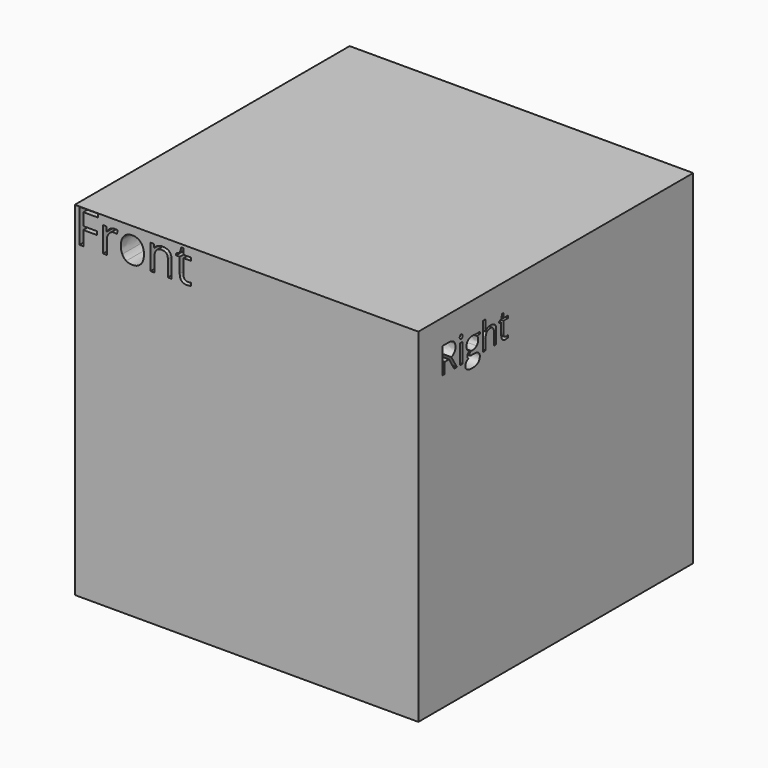
from build123d import *

# Parameters (mm, degrees)
F0_W     = 150
F0_H     = 150
F2_DEPTH = 75
F1_W     = 150
F1_H     = 150
F1_W_2   = 1.2864061088
F1_H_2   = 8.4892888683
F3_DEPTH = 75


with BuildPart() as f2:
    # F0 (on Front) → F2 (new body, symmetric)
    with BuildSketch(Plane.XZ):
        Rectangle(F0_W, F0_H)
        Polygon((-71.2858654449, 66.4917797723), (-71.2858654449, 60.2331906557), (-72.9875094904, 60.2331906557), (-72.9875094904, 74.8750204938), (-64.8253863567, 74.8750204938), (-64.8253863567, 73.3624480089), (-71.2858654449, 73.3624480089), (-71.2858654449, 68.0043522573), (-65.2163478889, 68.0043522573), (-65.2163478889, 66.4917797723), align=None, mode=Mode.SUBTRACT)
        with BuildLine():
            add(Edge.make_bspline(
                [(-59.537791865, 70.8292095569), (-58.6757537327, 71.410844951), (-57.6438716561, 71.410844951)],
                knots=[0, 0, 0, 1, 1, 1], degree=2))
            add(Edge.make_bspline(
                [(-57.6438716561, 71.410844951), (-56.9132222354, 71.410844951), (-56.3331891427, 71.2890700476)],
                knots=[0, 0, 0, 1, 1, 1], degree=2))
            Line((-56.3331891427, 71.2890700476), (-56.5639205387, 69.7476561382))
            add(Edge.make_bspline(
                [(-56.5639205387, 69.7476561382), (-57.2432963158, 69.8982724661), (-57.7656465595, 69.8982724661)],
                knots=[0, 0, 0, 1, 1, 1], degree=2))
            add(Edge.make_bspline(
                [(-57.7656465595, 69.8982724661), (-59.098761292, 69.8982724661), (-60.0441190951, 68.8167190474)],
                knots=[0, 0, 0, 1, 1, 1], degree=2))
            add(Edge.make_bspline(
                [(-60.0441190951, 68.8167190474), (-60.9894768982, 67.7351656286), (-60.9894768982, 66.1232504593)],
                knots=[0, 0, 0, 1, 1, 1], degree=2))
            Line((-60.9894768982, 66.1232504593), (-60.9894768982, 60.2331906557))
            Line((-60.9894768982, 60.2331906557), (-62.652665711, 60.2331906557))
            Line((-62.652665711, 60.2331906557), (-62.652665711, 71.2089549795))
            Line((-62.652665711, 71.2089549795), (-61.2810957459, 71.2089549795))
            Line((-61.2810957459, 71.2089549795), (-61.0888195826, 69.1772368536))
            Line((-61.0888195826, 69.1772368536), (-61.0087045145, 69.1772368536))
            add(Edge.make_bspline(
                [(-61.0087045145, 69.1772368536), (-60.3998299973, 70.2475741629), (-59.537791865, 70.8292095569)],
                knots=[0, 0, 0, 1, 1, 1], degree=2))
        make_face(mode=Mode.SUBTRACT)
        with BuildLine():
            add(Edge.make_bspline(
                [(-46.1633824035, 69.8774425484), (-44.8062331506, 68.3440401458), (-44.8062331506, 65.7322889272)],
                knots=[0, 0, 0, 1, 1, 1], degree=2))
            add(Edge.make_bspline(
                [(-44.8062331506, 65.7322889272), (-44.8062331506, 63.0468318459), (-46.1569731981, 61.539066265)],
                knots=[0, 0, 0, 1, 1, 1], degree=2))
            add(Edge.make_bspline(
                [(-46.1569731981, 61.539066265), (-47.5077132455, 60.0313006842), (-49.8919376709, 60.0313006842)],
                knots=[0, 0, 0, 1, 1, 1], degree=2))
            add(Edge.make_bspline(
                [(-49.8919376709, 60.0313006842), (-51.3660549231, 60.0313006842), (-52.5068934923, 60.7234948722)],
                knots=[0, 0, 0, 1, 1, 1], degree=2))
            add(Edge.make_bspline(
                [(-52.5068934923, 60.7234948722), (-53.6477320614, 61.4156890602), (-54.2694249895, 62.7071439573)],
                knots=[0, 0, 0, 1, 1, 1], degree=2))
            add(Edge.make_bspline(
                [(-54.2694249895, 62.7071439573), (-54.8911179177, 63.9985988544), (-54.8911179177, 65.7322889272)],
                knots=[0, 0, 0, 1, 1, 1], degree=2))
            add(Edge.make_bspline(
                [(-54.8911179177, 65.7322889272), (-54.8911179177, 68.4145414057), (-53.548389377, 69.9126931784)],
                knots=[0, 0, 0, 1, 1, 1], degree=2))
            add(Edge.make_bspline(
                [(-53.548389377, 69.9126931784), (-52.2056608364, 71.410844951), (-49.821436411, 71.410844951)],
                knots=[0, 0, 0, 1, 1, 1], degree=2))
            add(Edge.make_bspline(
                [(-49.821436411, 71.410844951), (-47.5205316564, 71.410844951), (-46.1633824035, 69.8774425484)],
                knots=[0, 0, 0, 1, 1, 1], degree=2))
        make_face(mode=Mode.SUBTRACT)
        with BuildLine():
            Line((-32.7152670794, 60.2331906557), (-34.3784558923, 60.2331906557))
            Line((-34.3784558923, 60.2331906557), (-34.3784558923, 67.3345902883))
            add(Edge.make_bspline(
                [(-34.3784558923, 67.3345902883), (-34.3784558923, 68.6741142262), (-34.9889327109, 69.3358646884)],
                knots=[0, 0, 0, 1, 1, 1], degree=2))
            add(Edge.make_bspline(
                [(-34.9889327109, 69.3358646884), (-35.5994095295, 69.9976151505), (-36.9036828375, 69.9976151505)],
                knots=[0, 0, 0, 1, 1, 1], degree=2))
            add(Edge.make_bspline(
                [(-36.9036828375, 69.9976151505), (-38.6245544993, 69.9976151505), (-39.4257051799, 69.0666780597)],
                knots=[0, 0, 0, 1, 1, 1], degree=2))
            add(Edge.make_bspline(
                [(-39.4257051799, 69.0666780597), (-40.2268558605, 68.1357409689), (-40.2268558605, 65.9918617477)],
                knots=[0, 0, 0, 1, 1, 1], degree=2))
            Line((-40.2268558605, 65.9918617477), (-40.2268558605, 60.2331906557))
            Line((-40.2268558605, 60.2331906557), (-41.8900446733, 60.2331906557))
            Line((-41.8900446733, 60.2331906557), (-41.8900446733, 71.2089549795))
            Line((-41.8900446733, 71.2089549795), (-40.5377023245, 71.2089549795))
            Line((-40.5377023245, 71.2089549795), (-40.2685156959, 69.7059963028))
            Line((-40.2685156959, 69.7059963028), (-40.1884006278, 69.7059963028))
            add(Edge.make_bspline(
                [(-40.1884006278, 69.7059963028), (-39.6756641922, 70.5167607915), (-38.7543409096, 70.9638028713)],
                knots=[0, 0, 0, 1, 1, 1], degree=2))
            add(Edge.make_bspline(
                [(-38.7543409096, 70.9638028713), (-37.8330176269, 71.410844951), (-36.701792866, 71.410844951)],
                knots=[0, 0, 0, 1, 1, 1], degree=2))
            add(Edge.make_bspline(
                [(-36.701792866, 71.410844951), (-34.7181437809, 71.410844951), (-33.7167054302, 70.4542710384)],
                knots=[0, 0, 0, 1, 1, 1], degree=2))
            add(Edge.make_bspline(
                [(-33.7167054302, 70.4542710384), (-32.7152670794, 69.4976971258), (-32.7152670794, 67.3922731373)],
                knots=[0, 0, 0, 1, 1, 1], degree=2))
            Line((-32.7152670794, 67.3922731373), (-32.7152670794, 60.2331906557))
        make_face(mode=Mode.SUBTRACT)
        with BuildLine():
            add(Edge.make_bspline(
                [(-27.0495294664, 61.9364370026), (-26.5784528663, 61.4060752521), (-25.7580745694, 61.4060752521)],
                knots=[0, 0, 0, 1, 1, 1], degree=2))
            add(Edge.make_bspline(
                [(-25.7580745694, 61.4060752521), (-25.3158393937, 61.4060752521), (-24.9056502452, 61.4701673065)],
                knots=[0, 0, 0, 1, 1, 1], degree=2))
            add(Edge.make_bspline(
                [(-24.9056502452, 61.4701673065), (-24.4954610968, 61.534259361), (-24.2551158926, 61.6047606208)],
                knots=[0, 0, 0, 1, 1, 1], degree=2))
            Line((-24.2551158926, 61.6047606208), (-24.2551158926, 60.3325333401))
            add(Edge.make_bspline(
                [(-24.2551158926, 60.3325333401), (-24.5243025213, 60.2043492312), (-25.0498573677, 60.1178249577)],
                knots=[0, 0, 0, 1, 1, 1], degree=2))
            add(Edge.make_bspline(
                [(-25.0498573677, 60.1178249577), (-25.5754122142, 60.0313006842), (-25.9984197735, 60.0313006842)],
                knots=[0, 0, 0, 1, 1, 1], degree=2))
            add(Edge.make_bspline(
                [(-25.9984197735, 60.0313006842), (-29.1805902768, 60.0313006842), (-29.1805902768, 63.3865197344)],
                knots=[0, 0, 0, 1, 1, 1], degree=2))
            Line((-29.1805902768, 63.3865197344), (-29.1805902768, 69.9175000825))
            Line((-29.1805902768, 69.9175000825), (-30.7540502134, 69.9175000825))
            Line((-30.7540502134, 69.9175000825), (-30.7540502134, 70.718650763))
            Line((-30.7540502134, 70.718650763), (-29.1805902768, 71.410844951))
            Line((-29.1805902768, 71.410844951), (-28.4819868833, 73.753409541))
            Line((-28.4819868833, 73.753409541), (-27.5206060666, 73.753409541))
            Line((-27.5206060666, 73.753409541), (-27.5206060666, 71.2089549795))
            Line((-27.5206060666, 71.2089549795), (-24.3352309607, 71.2089549795))
            Line((-24.3352309607, 71.2089549795), (-24.3352309607, 69.9175000825))
            Line((-24.3352309607, 69.9175000825), (-27.5206060666, 69.9175000825))
            Line((-27.5206060666, 69.9175000825), (-27.5206060666, 63.4570209943))
            add(Edge.make_bspline(
                [(-27.5206060666, 63.4570209943), (-27.5206060666, 62.4667987531), (-27.0495294664, 61.9364370026)],
                knots=[0, 0, 0, 1, 1, 1], degree=2))
        make_face(mode=Mode.SUBTRACT)
    extrude(amount=F2_DEPTH, both=True)

    # F1 (on Right) → F3 (intersect, symmetric)
    with BuildSketch(Plane.YZ):
        Rectangle(F1_W, F1_H)
        with BuildLine():
            Line((-44.2826830679, 61.3081981557), (-41.3479916751, 61.3081981557))
            Line((-41.3479916751, 61.3081981557), (-41.3479916751, 60.495209324))
            Line((-41.3479916751, 60.495209324), (-42.9194396, 60.3093124874))
            add(Edge.make_bspline(
                [(-42.9194396, 60.3093124874), (-42.7037992696, 60.0391424183), (-42.53277418, 59.6004258841)],
                knots=[0, 0, 0, 1, 1, 1], degree=2))
            add(Edge.make_bspline(
                [(-42.53277418, 59.6004258841), (-42.3617490904, 59.1617093499), (-42.3617490904, 58.6139333383)],
                knots=[0, 0, 0, 1, 1, 1], degree=2))
            add(Edge.make_bspline(
                [(-42.3617490904, 58.6139333383), (-42.3617490904, 57.3647065968), (-43.2143959139, 56.6211192506)],
                knots=[0, 0, 0, 1, 1, 1], degree=2))
            add(Edge.make_bspline(
                [(-43.2143959139, 56.6211192506), (-44.0670427375, 55.8775319045), (-45.5542174297, 55.8775319045)],
                knots=[0, 0, 0, 1, 1, 1], degree=2))
            add(Edge.make_bspline(
                [(-45.5542174297, 55.8775319045), (-45.9334469763, 55.8775319045), (-46.2655826575, 55.9394975167)],
                knots=[0, 0, 0, 1, 1, 1], degree=2))
            add(Edge.make_bspline(
                [(-46.2655826575, 55.9394975167), (-47.0860073627, 55.5057382315), (-47.0860073627, 54.8489027424)],
                knots=[0, 0, 0, 1, 1, 1], degree=2))
            add(Edge.make_bspline(
                [(-47.0860073627, 54.8489027424), (-47.0860073627, 54.4994166897), (-46.7997262345, 54.3333488491)],
                knots=[0, 0, 0, 1, 1, 1], degree=2))
            add(Edge.make_bspline(
                [(-46.7997262345, 54.3333488491), (-46.5134451062, 54.1672810084), (-45.8169516254, 54.1672810084)],
                knots=[0, 0, 0, 1, 1, 1], degree=2))
            Line((-45.8169516254, 54.1672810084), (-44.3149051862, 54.1672810084))
            add(Edge.make_bspline(
                [(-44.3149051862, 54.1672810084), (-42.9343113469, 54.1672810084), (-42.1956812497, 53.5860435662)],
                knots=[0, 0, 0, 1, 1, 1], degree=2))
            add(Edge.make_bspline(
                [(-42.1956812497, 53.5860435662), (-41.4570511526, 53.004806124), (-41.4570511526, 51.8968609783)],
                knots=[0, 0, 0, 1, 1, 1], degree=2))
            add(Edge.make_bspline(
                [(-41.4570511526, 51.8968609783), (-41.4570511526, 50.4865236451), (-42.5873039187, 49.7466542357)],
                knots=[0, 0, 0, 1, 1, 1], degree=2))
            add(Edge.make_bspline(
                [(-42.5873039187, 49.7466542357), (-43.7175566848, 49.0067848263), (-45.886353111, 49.0067848263)],
                knots=[0, 0, 0, 1, 1, 1], degree=2))
            add(Edge.make_bspline(
                [(-45.886353111, 49.0067848263), (-47.5519887663, 49.0067848263), (-48.4542080796, 49.6264409481)],
                knots=[0, 0, 0, 1, 1, 1], degree=2))
            add(Edge.make_bspline(
                [(-48.4542080796, 49.6264409481), (-49.3564273929, 50.2460970699), (-49.3564273929, 51.3788284605)],
                knots=[0, 0, 0, 1, 1, 1], degree=2))
            add(Edge.make_bspline(
                [(-49.3564273929, 51.3788284605), (-49.3564273929, 52.1521593004), (-48.8607024955, 52.7185249957)],
                knots=[0, 0, 0, 1, 1, 1], degree=2))
            add(Edge.make_bspline(
                [(-48.8607024955, 52.7185249957), (-48.3649775981, 53.284890691), (-47.4677155338, 53.4856592745)],
                knots=[0, 0, 0, 1, 1, 1], degree=2))
            add(Edge.make_bspline(
                [(-47.4677155338, 53.4856592745), (-47.7924153416, 53.6318981192), (-48.0130129209, 53.9417261801)],
                knots=[0, 0, 0, 1, 1, 1], degree=2))
            add(Edge.make_bspline(
                [(-48.0130129209, 53.9417261801), (-48.2336105003, 54.251554241), (-48.2336105003, 54.6630059058)],
                knots=[0, 0, 0, 1, 1, 1], degree=2))
            add(Edge.make_bspline(
                [(-48.2336105003, 54.6630059058), (-48.2336105003, 55.1265086849), (-47.9857480516, 55.4759947376)],
                knots=[0, 0, 0, 1, 1, 1], degree=2))
            add(Edge.make_bspline(
                [(-47.9857480516, 55.4759947376), (-47.7378856029, 55.8254807903), (-47.2025027136, 56.1501805981)],
                knots=[0, 0, 0, 1, 1, 1], degree=2))
            add(Edge.make_bspline(
                [(-47.2025027136, 56.1501805981), (-47.8618168272, 56.4203506672), (-48.2757471166, 57.0709895951)],
                knots=[0, 0, 0, 1, 1, 1], degree=2))
            add(Edge.make_bspline(
                [(-48.2757471166, 57.0709895951), (-48.6896774059, 57.7216285229), (-48.6896774059, 58.5594035996)],
                knots=[0, 0, 0, 1, 1, 1], degree=2))
            add(Edge.make_bspline(
                [(-48.6896774059, 58.5594035996), (-48.6896774059, 59.9523905613), (-47.8531416415, 60.7083710299)],
                knots=[0, 0, 0, 1, 1, 1], degree=2))
            add(Edge.make_bspline(
                [(-47.8531416415, 60.7083710299), (-47.0166058771, 61.4643514984), (-45.4848159441, 61.4643514984)],
                knots=[0, 0, 0, 1, 1, 1], degree=2))
            add(Edge.make_bspline(
                [(-45.4848159441, 61.4643514984), (-44.8180659571, 61.4643514984), (-44.2826830679, 61.3081981557)],
                knots=[0, 0, 0, 1, 1, 1], degree=2))
        make_face(mode=Mode.SUBTRACT)
        with BuildLine():
            Line((-58.2398175546, 57.5282958129), (-60.6044253153, 57.5282958129))
            Line((-60.6044253153, 57.5282958129), (-60.6044253153, 52.8189092875))
            Line((-60.6044253153, 52.8189092875), (-61.920574918, 52.8189092875))
            Line((-61.920574918, 52.8189092875), (-61.920574918, 64.143744569))
            Line((-61.920574918, 64.143744569), (-58.8148584357, 64.143744569))
            add(Edge.make_bspline(
                [(-58.8148584357, 64.143744569), (-56.730335242, 64.143744569), (-55.7351675104, 63.3456274841)],
                knots=[0, 0, 0, 1, 1, 1], degree=2))
            add(Edge.make_bspline(
                [(-55.7351675104, 63.3456274841), (-54.7399997789, 62.5475103993), (-54.7399997789, 60.9438403561)],
                knots=[0, 0, 0, 1, 1, 1], degree=2))
            add(Edge.make_bspline(
                [(-54.7399997789, 60.9438403561), (-54.7399997789, 58.6982065708), (-57.0178556825, 57.9075253594)],
                knots=[0, 0, 0, 1, 1, 1], degree=2))
            Line((-57.0178556825, 57.9075253594), (-53.941882694, 52.8189092875))
            Line((-53.941882694, 52.8189092875), (-55.4984588719, 52.8189092875))
            Line((-55.4984588719, 52.8189092875), (-58.2398175546, 57.5282958129))
        make_face(mode=Mode.SUBTRACT)
        with Locations((-51.6652661026, 57.0635537216)):
            Rectangle(F1_W_2, F1_H_2, mode=Mode.SUBTRACT)
        with BuildLine():
            add(Edge.make_bspline(
                [(-52.2006489919, 62.9614406886), (-52.4175286345, 63.1746023945), (-52.4175286345, 63.6083616798)],
                knots=[0, 0, 0, 1, 1, 1], degree=2))
            add(Edge.make_bspline(
                [(-52.4175286345, 63.6083616798), (-52.4175286345, 64.0495568385), (-52.2006489919, 64.2552826709)],
                knots=[0, 0, 0, 1, 1, 1], degree=2))
            add(Edge.make_bspline(
                [(-52.2006489919, 64.2552826709), (-51.9837693492, 64.4610085033), (-51.6565909169, 64.4610085033)],
                knots=[0, 0, 0, 1, 1, 1], degree=2))
            add(Edge.make_bspline(
                [(-51.6565909169, 64.4610085033), (-51.3467628561, 64.4610085033), (-51.12244734, 64.2515647341)],
                knots=[0, 0, 0, 1, 1, 1], degree=2))
            add(Edge.make_bspline(
                [(-51.12244734, 64.2515647341), (-50.8981318239, 64.042120965), (-50.8981318239, 63.6083616798)],
                knots=[0, 0, 0, 1, 1, 1], degree=2))
            add(Edge.make_bspline(
                [(-50.8981318239, 63.6083616798), (-50.8981318239, 63.1746023945), (-51.12244734, 62.9614406886)],
                knots=[0, 0, 0, 1, 1, 1], degree=2))
            add(Edge.make_bspline(
                [(-51.12244734, 62.9614406886), (-51.3467628561, 62.7482789827), (-51.6565909169, 62.7482789827)],
                knots=[0, 0, 0, 1, 1, 1], degree=2))
            add(Edge.make_bspline(
                [(-51.6565909169, 62.7482789827), (-51.9837693492, 62.7482789827), (-52.2006489919, 62.9614406886)],
                knots=[0, 0, 0, 1, 1, 1], degree=2))
        make_face(mode=Mode.SUBTRACT)
        with BuildLine():
            Line((-32.5092167542, 52.8189092875), (-33.795622863, 52.8189092875))
            Line((-33.795622863, 52.8189092875), (-33.795622863, 58.3115411508))
            add(Edge.make_bspline(
                [(-33.795622863, 58.3115411508), (-33.795622863, 59.3476061864), (-34.2678008278, 59.859442143)],
                knots=[0, 0, 0, 1, 1, 1], degree=2))
            add(Edge.make_bspline(
                [(-34.2678008278, 59.859442143), (-34.7399787926, 60.3712780996), (-35.7487789588, 60.3712780996)],
                knots=[0, 0, 0, 1, 1, 1], degree=2))
            add(Edge.make_bspline(
                [(-35.7487789588, 60.3712780996), (-37.0872361818, 60.3712780996), (-37.7031743669, 59.6425625004)],
                knots=[0, 0, 0, 1, 1, 1], degree=2))
            add(Edge.make_bspline(
                [(-37.7031743669, 59.6425625004), (-38.3191125519, 58.9138469012), (-38.3191125519, 57.2581257438)],
                knots=[0, 0, 0, 1, 1, 1], degree=2))
            Line((-38.3191125519, 57.2581257438), (-38.3191125519, 52.8189092875))
            Line((-38.3191125519, 52.8189092875), (-39.6055186607, 52.8189092875))
            Line((-39.6055186607, 52.8189092875), (-39.6055186607, 64.8724601682))
            Line((-39.6055186607, 64.8724601682), (-38.3191125519, 64.8724601682))
            Line((-38.3191125519, 64.8724601682), (-38.3191125519, 61.2239249232))
            add(Edge.make_bspline(
                [(-38.3191125519, 61.2239249232), (-38.3191125519, 60.5646108096), (-38.3810781641, 60.1308515244)],
                knots=[0, 0, 0, 1, 1, 1], degree=2))
            Line((-38.3810781641, 60.1308515244), (-38.304240805, 60.1308515244))
            add(Edge.make_bspline(
                [(-38.304240805, 60.1308515244), (-37.9250112585, 60.7430717727), (-37.2235605286, 61.0950364498)],
                knots=[0, 0, 0, 1, 1, 1], degree=2))
            add(Edge.make_bspline(
                [(-37.2235605286, 61.0950364498), (-36.5221097988, 61.447001127), (-35.6248477345, 61.447001127)],
                knots=[0, 0, 0, 1, 1, 1], degree=2))
            add(Edge.make_bspline(
                [(-35.6248477345, 61.447001127), (-34.0682715566, 61.447001127), (-33.2887441554, 60.7071317176)],
                knots=[0, 0, 0, 1, 1, 1], degree=2))
            add(Edge.make_bspline(
                [(-33.2887441554, 60.7071317176), (-32.5092167542, 59.9672623082), (-32.5092167542, 58.3561563916)],
                knots=[0, 0, 0, 1, 1, 1], degree=2))
            Line((-32.5092167542, 58.3561563916), (-32.5092167542, 52.8189092875))
        make_face(mode=Mode.SUBTRACT)
        with BuildLine():
            add(Edge.make_bspline(
                [(-28.127008661, 54.1362982023), (-27.7626508614, 53.7260858497), (-27.1281229927, 53.7260858497)],
                knots=[0, 0, 0, 1, 1, 1], degree=2))
            add(Edge.make_bspline(
                [(-27.1281229927, 53.7260858497), (-26.7860728135, 53.7260858497), (-26.4688088791, 53.7756583395)],
                knots=[0, 0, 0, 1, 1, 1], degree=2))
            add(Edge.make_bspline(
                [(-26.4688088791, 53.7756583395), (-26.1515449448, 53.8252308292), (-25.9656481083, 53.8797605679)],
                knots=[0, 0, 0, 1, 1, 1], degree=2))
            Line((-25.9656481083, 53.8797605679), (-25.9656481083, 52.8957466466))
            add(Edge.make_bspline(
                [(-25.9656481083, 52.8957466466), (-26.1738525652, 52.7966016671), (-26.5803469811, 52.7296788059)],
                knots=[0, 0, 0, 1, 1, 1], degree=2))
            add(Edge.make_bspline(
                [(-26.5803469811, 52.7296788059), (-26.9868413969, 52.6627559448), (-27.3140198292, 52.6627559448)],
                knots=[0, 0, 0, 1, 1, 1], degree=2))
            add(Edge.make_bspline(
                [(-27.3140198292, 52.6627559448), (-29.7752939449, 52.6627559448), (-29.7752939449, 55.2578757827)],
                knots=[0, 0, 0, 1, 1, 1], degree=2))
            Line((-29.7752939449, 55.2578757827), (-29.7752939449, 60.3093124874))
            Line((-29.7752939449, 60.3093124874), (-30.9922985681, 60.3093124874))
            Line((-30.9922985681, 60.3093124874), (-30.9922985681, 60.9289686092))
            Line((-30.9922985681, 60.9289686092), (-29.7752939449, 61.4643514984))
            Line((-29.7752939449, 61.4643514984), (-29.2349538067, 63.2762259985))
            Line((-29.2349538067, 63.2762259985), (-28.4913664606, 63.2762259985))
            Line((-28.4913664606, 63.2762259985), (-28.4913664606, 61.3081981557))
            Line((-28.4913664606, 61.3081981557), (-26.0276137204, 61.3081981557))
            Line((-26.0276137204, 61.3081981557), (-26.0276137204, 60.3093124874))
            Line((-26.0276137204, 60.3093124874), (-28.4913664606, 60.3093124874))
            Line((-28.4913664606, 60.3093124874), (-28.4913664606, 55.3124055215))
            add(Edge.make_bspline(
                [(-28.4913664606, 55.3124055215), (-28.4913664606, 54.546510555), (-28.127008661, 54.1362982023)],
                knots=[0, 0, 0, 1, 1, 1], degree=2))
        make_face(mode=Mode.SUBTRACT)
    extrude(amount=F3_DEPTH, both=True, mode=Mode.INTERSECT)


solid = f2.part
